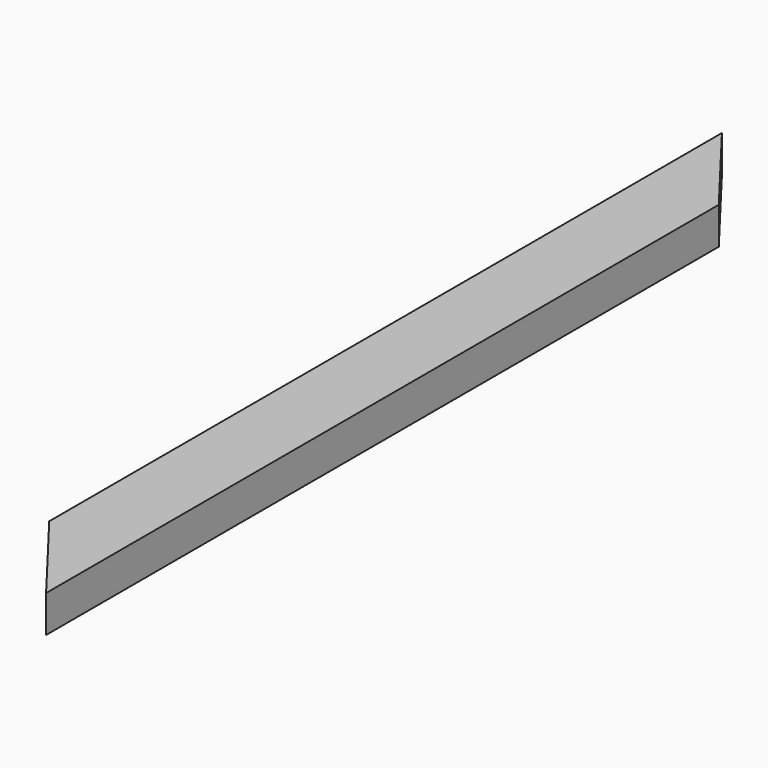
from build123d import *

# Parameters (mm, degrees)
F0_W     = 38.1
F0_H     = 19.05
F1_DEPTH = 508
F3_DEPTH = 19.051


# Not quite as in the source:
# - a feature names something its author has since deleted; it is built from what else it names


with BuildPart() as f1:
    # F0 (on Front) → F1 (new body)
    with BuildSketch(Plane.XZ):
        Rectangle(F0_W, F0_H)
    extrude(amount=F1_DEPTH)

    # F2 (on face) → F3 (cut, through all)
    with BuildSketch(Plane.XY.offset(9.525)):
        Polygon((19.05, 0), (-19.05, 0), (19.05, -49.6528867052), align=None)
        Polygon((19.05, -483.0208308118), (-19.05, -433.3679441065), (-19.05, -508), (19.05, -508), align=None)
    extrude(amount=-F3_DEPTH, mode=Mode.SUBTRACT)


solid = f1.part
